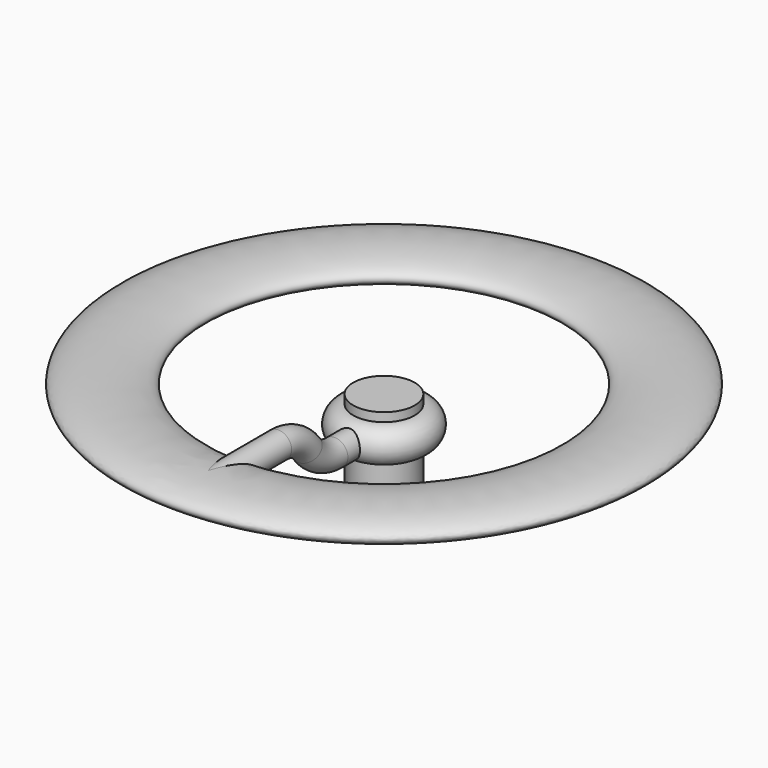
from build123d import *

# Parameters (mm, degrees)
F5_R = 15


with BuildPart() as f1:
    # F0 (on Front) → F1 (revolve)
    with BuildSketch(Plane.XZ):
        with BuildLine():
            Line((-35, 0), (0, 0))
            Line((0, 0), (0, 100))
            Line((0, 100), (-35, 100))
            Line((-35, 100), (-35, 90))
            ThreePointArc((-35, 90), (-55, 70), (-35, 50))
            Line((-35, 50), (-35, 0))
        make_face()
    revolve(axis=Axis((0, 0, 50), (0, 0, 1)))



with BuildPart() as f3:
    # F2 (on Right) → F3 (revolve)
    with BuildSketch(Plane.YZ):
        with BuildLine():
            add(Edge.make_bspline(
                [(-200, 110), (-200, 135.980762), (-275, 122.990381), (-350, 110), (-275, 97.009619), (-200, 84.019238), (-200, 110)],
                knots=[0, 0, 0, 2.094395, 2.094395, 4.18879, 4.18879, 6.283185, 6.283185, 6.283185], degree=2, weights=[1, 0.5, 1, 0.5, 1, 0.5, 1]))
        make_face()
    revolve(axis=Axis((0, 0, 68.003841), (0, 0, 1)))


with BuildPart() as f1_1:
    add(f1.part)

    add(f3.part)  # F6 merges F3
    # F6: sweep along a path in F4
    with BuildLine(Plane.YZ) as f6_path:
        Line((-250, 110), (-150, 110))
        ThreePointArc((-150, 110), (-127.63932, 104.72136), (-110, 90))
        ThreePointArc((-110, 90), (-92.36068, 75.27864), (-70, 70))
        Line((-70, 70), (0, 70))
    # F5 (on Front) → F6 (sweep)
    with BuildSketch(Plane.XZ):
        with Locations((0, 70)):
            Circle(F5_R)
    sweep(path=f6_path.line)


solid = f1_1.part
